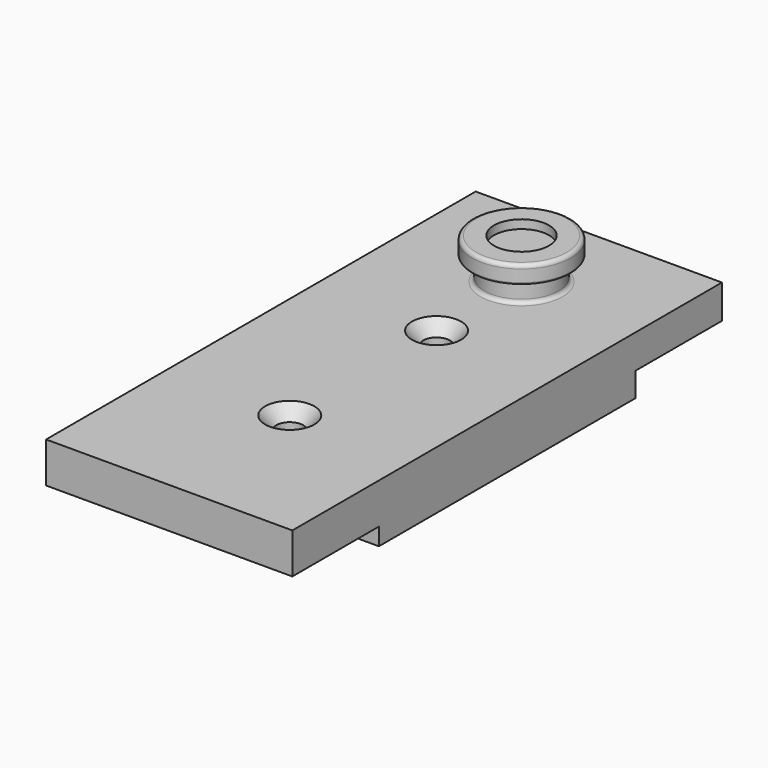
from build123d import *

# Parameters (mm, degrees)
F2_R            = 0.508
F3_S5_R         = 4.8895
F3_T6_DEPTH     = 11
F4_R            = 0.254
F5_W            = 70.612
F5_H            = 7.62
F6_DEPTH        = 16.1925
F7_W            = 14.224
F7_H            = 3.175
F7_H_2          = 2.286
F8_DEPTH        = 32.386
F10_D           = 3.5179
F10_CSINK_D     = 6.477
F10_CSINK_ANGLE = 82


# Not quite as in the source:
# - a fillet or chamfer that OpenCascade refuses, or shapes differently, is made with other operations: its cross-section is extruded or revolved along the edge and cut away or added


with BuildPart() as f1:
    # F0 (on Front) → F1 (revolve)
    with BuildSketch(Plane.XZ):
        Polygon((0, 9.271), (0, 0), (11.1125, 0), (11.1125, 5.08), (4.8895, 5.08), (4.8895, 7.62), (6.477, 7.62), (6.477, 10.414), (3.6195, 10.414), (3.6195, 9.271), align=None)
    revolve(axis=Axis((0, 0, 5.207), (0, 0, -1)))

    # F2
    f2_edges = [f1.edges().sort_by_distance(p)[0] for p in [
        (-6.477, 0, 10.414),
        (-4.8895, 0, 5.08),
    ]]
    fillet(f2_edges, radius=F2_R)

    # F3: chamfer of 0.508 x 1.5917743649 on 1 edges, made by hand


with BuildPart() as f3_tool2:
    # F3_s3 → F3_t4 (revolve)
    with BuildSketch(Plane.XZ):
        Polygon((4.8852256351, 7.62), (6.477, 8.128), (6.477, 7.62), align=None)
    revolve(axis=Axis((0, 0, 7.62), (0, 0, -1)))

    # F3_s5 → F3_t6 (cut, symmetric)
    with BuildSketch(Plane.XY.offset(7.9)):
        Circle(F3_S5_R)
    extrude(amount=F3_T6_DEPTH, both=True, mode=Mode.SUBTRACT)


with BuildPart() as f1_1:
    add(f1.part)

    # F3_t1: cut F3_tool2
    add(f3_tool2.part, mode=Mode.SUBTRACT)

    # F4
    f4_edges = [f1_1.edges().sort_by_distance(p)[0] for p in [
        (-6.477, 0, 8.128),
    ]]
    fillet(f4_edges, radius=F4_R)

    # F5 (on Right) → F6 (join, symmetric)
    with BuildSketch(Plane.YZ):
        with Locations((-22.606, 1.27)):
            Rectangle(F5_W, F5_H)
    extrude(amount=F6_DEPTH, both=True)

    # F7 (on face) → F8 (cut, through all)
    with BuildSketch(Plane(origin=(-16.1925, 0, 0), x_dir=(0, -1, 0), z_dir=(-1, 0, 0))):
        with Locations((-5.588, -0.9525)):
            Rectangle(F7_W, F7_H)
        with Locations((50.8, -1.397)):
            Rectangle(F7_W, F7_H_2)
    extrude(amount=-F8_DEPTH, mode=Mode.SUBTRACT)

    # F10 (through all)
    with Locations(Plane.XY.offset(5.08)):
        with Locations((0, -13.97), (0, -38.1)):
            CounterSinkHole(F10_D / 2, F10_CSINK_D / 2, counter_sink_angle=F10_CSINK_ANGLE)


solid = f1_1.part
